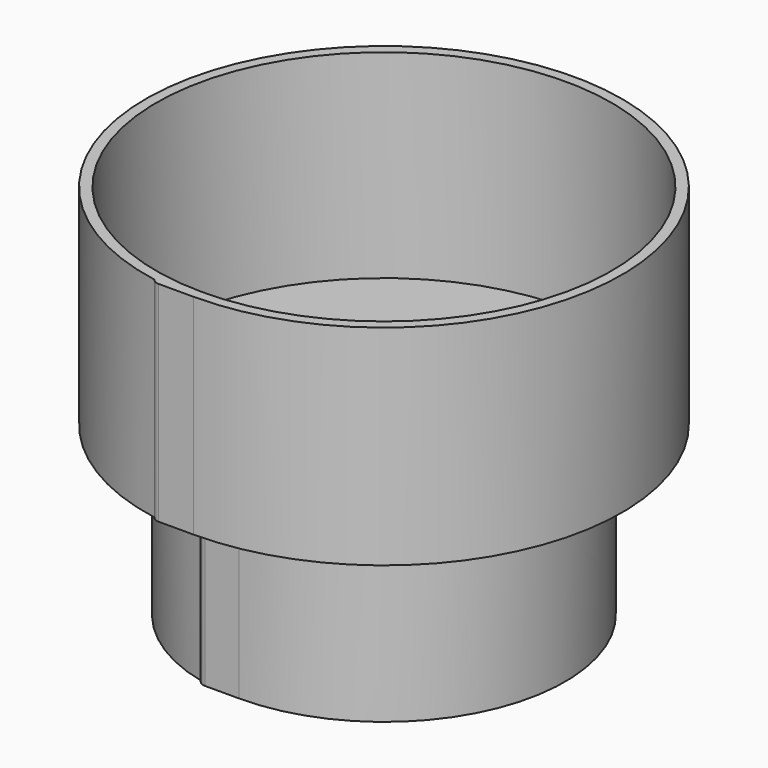
from build123d import *

# Parameters (mm, degrees)
F1_DEPTH    = 25.4
F3_T1_DEPTH = 113.1592478003
F3_T3_DEPTH = 148.0952074612


# Not quite as in the source:
# - a fillet or chamfer that OpenCascade refuses, or shapes differently, is made with other operations: its cross-section is extruded or revolved along the edge and cut away or added


with BuildPart() as f1:
    # F0 (on Right) → F1 (new body)
    with BuildSketch(Plane.YZ):
        Polygon((-103.5402726054, 0), (0, 0), (0, 6.35), (-138.112494323, 6.35), (-138.112494323, 127), (-144.462494323, 127), (-144.462494323, 0), (-109.8902726054, 0), align=None)
        Polygon((-103.5402726054, -95.25), (-103.5402726054, 0), (-109.8902726054, 0), (-109.8902726054, -101.6), (0, -101.6), (0, -95.25), align=None)
    extrude(amount=F1_DEPTH)

    # F1_face (on face) → F2 (revolve)
    with BuildSketch(Plane(origin=(25.4, -92.8938883884, -14.564984288), x_dir=(0, 1, 0), z_dir=(1, 0, 0))):
        Polygon((-51.5686059346, 14.564984288), (-16.996384217, 14.564984288), (-16.996384217, -87.035015712), (92.8938883884, -87.035015712), (92.8938883884, -80.685015712), (-10.646384217, -80.685015712), (-10.646384217, 14.564984288), (92.8938883884, 14.564984288), (92.8938883884, 20.914984288), (-45.2186059346, 20.914984288), (-45.2186059346, 141.564984288), (-51.5686059346, 141.564984288), align=None)
    revolve(axis=Axis((25.4, 0, 3.175), (0, 0, -1)))

    # F3: fillet of radius 5.08 on 4 edges, made by hand

    # F3_s2 → F3_t1 (cut)
    with BuildSketch(Plane.XY.offset(-113.1592478003)):
        with BuildLine():
            ThreePointArc((0, -106.9145079645), (1.8744370031, -109.0820354513), (4.6236991201, -109.8902726054))
            Line((4.6236991201, -109.8902726054), (4.6236991201, -109.9918726054))
            Line((4.6236991201, -109.9918726054), (0, -109.9918726054))
            Line((0, -109.9918726054), (-0.1016, -109.8902726054))
            ThreePointArc((-0.1016, -109.8902726054), (-0.1016, -108.4023902849), (-0.0924739824, -106.9565926716))
            Line((-0.0924739824, -106.9565926716), (0, -106.9145079645))
        make_face()
    extrude(amount=F3_T1_DEPTH, mode=Mode.SUBTRACT)

    # F3_s4 → F3_t3 (cut)
    with BuildSketch(Plane.XY.offset(-10.5476037306)):
        with BuildLine():
            ThreePointArc((4.2190414922, -144.462494323), (1.8281710158, -143.8646967241), (0, -142.2119976163))
            Line((0, -142.2119976163), (-0.0843808298, -142.2685876821))
            ThreePointArc((-0.0843808298, -142.2685876821), (-0.1016, -143.3372459696), (-0.1016, -144.462494323))
            Line((-0.1016, -144.462494323), (0, -144.564094323))
            Line((0, -144.564094323), (4.2190414922, -144.564094323))
            Line((4.2190414922, -144.564094323), (4.2190414922, -144.462494323))
        make_face()
    extrude(amount=F3_T3_DEPTH, mode=Mode.SUBTRACT)


solid = f1.part
